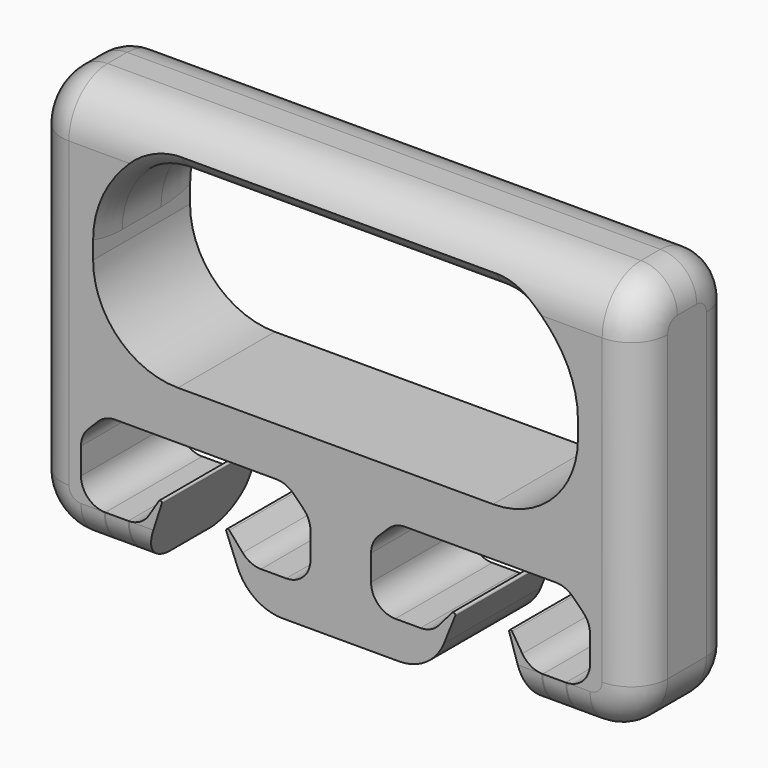
from build123d import *

# Parameters (mm, degrees)
F0_W        = 101.6
F0_H        = 38.1
F0_W_2      = 12.7
F0_H_2      = 7.6156796026
F1_DEPTH    = 25.4
F2_F1_R     = 0.3302
F2_F2_R     = 0.3302
F3_R        = 5.08
F5_R        = 10.15999
F6_T1_DEPTH = 101.6
F8_R        = 7.62
F9_W        = 12.7
F9_H        = 7.62
F10_DEPTH   = 25.4
F11_F1_R    = 0.381
F11_F2_R    = 0.381
F12_R       = 5.08
F13_SIZE    = 5.08
F14_R       = 5.08
F15_R       = 17.78
F16_R       = 10.16


# Not quite as in the source:
# - a fillet or chamfer that OpenCascade refuses, or shapes differently, is made with other operations: its cross-section is extruded or revolved along the edge and cut away or added
# - two fillets or chamfers of one size are made in one step
# - a fillet or chamfer is up to 0.001 mm smaller than in the source, because OpenCascade refuses the exact size


with BuildPart() as f1:
    # F0 (on Front) → F1 (new body)
    with BuildSketch(Plane.XZ):
        Polygon((63.5, 29.21), (-63.5, 29.21), (-63.5, -29.21), (-53.34, -29.21), (-5.08, -29.21), (-5.08, -29.2056796026), (5.08, -29.2056796026), (5.08, -29.21), (53.34, -29.21), (63.5, -29.21), align=None)
        Rectangle(F0_W, F0_H, mode=Mode.SUBTRACT)
        Polygon((63.5, -54.61), (63.5, -29.21), (53.34, -29.21), (53.34, -46.9943203974), (53.34, -54.61), align=None)
        with Locations((46.99, -50.8021601987)):
            Rectangle(F0_W_2, F0_H_2)
        Polygon((40.64, -54.61), (40.64, -46.9943203974), (35.5896614492, -38.9685556293), align=None)
        Polygon((-53.34, -29.21), (-63.5, -29.21), (-63.5, -54.61), (-53.34, -54.61), (-53.34, -46.9943203974), align=None)
        with Locations((-46.99, -50.8021601987)):
            Rectangle(F0_W_2, F0_H_2)
        Polygon((-35.5896614492, -38.9685556293), (-40.64, -46.9943203974), (-40.64, -54.61), align=None)
    extrude(amount=F1_DEPTH)

    # F2: fillet of radius 0.3302 on 2 edges, made by hand

    # F2_f1
    f2_f1_edges = [f1.edges().sort_by_distance(p)[0] for p in [
        (-35.5896614492, -12.7, -38.9685556293),
    ]]
    fillet(f2_f1_edges, radius=F2_F1_R)

    # F2_f2
    f2_f2_edges = [f1.edges().sort_by_distance(p)[0] for p in [
        (35.5896614492, -12.7, -38.9685556293),
    ]]
    fillet(f2_f2_edges, radius=F2_F2_R)

    # F3
    f3_edges = [f1.edges().sort_by_distance(p)[0] for p in [
        (53.34, -12.7, -46.99432),
        (-53.34, -12.7, -46.99432),
        (40.64, -12.7, -46.99432),
        (-40.64, -12.7, -46.99432),
    ]]
    fillet(f3_edges, radius=F3_R)

    # F5 (radius 10.16 in the source; OpenCascade refuses exactly that, so slightly less here)
    f5_edges = [f1.edges().sort_by_distance(p)[0] for p in [
        (-63.5, -12.7, -54.61),
        (63.5, -12.7, -54.61),
        (0, 0, 29.21),
        (0, -25.4, 29.21),
    ]]
    fillet(f5_edges, radius=F5_R)

    # F6: fillet of radius 7.62 on 2 edges, made by hand

    # F6_s2 → F6_t1 (cut)
    with BuildSketch(Plane.YZ.offset(-50.8)):
        with BuildLine():
            ThreePointArc((0, 26.67), (-2.2318463274, 21.2818463274), (-7.62, 19.05))
            Line((-7.62, 19.05), (0, 19.05))
            Line((0, 19.05), (0, 26.67))
        make_face()
        with BuildLine():
            ThreePointArc((-17.78, 19.05), (-23.1681536726, 21.2818463274), (-25.4, 26.67))
            Line((-25.4, 26.67), (-25.4, 19.05))
            Line((-25.4, 19.05), (-17.78, 19.05))
        make_face()
    extrude(amount=F6_T1_DEPTH, mode=Mode.SUBTRACT)

    # F8
    f8_edges = [f1.edges().sort_by_distance(p)[0] for p in [
        (-63.5, -25.4, -12.7),
        (-63.5, 0, -12.7),
        (63.5, 0, -12.7),
        (63.5, -25.4, -12.7),
        (46.990005, 0, -54.61),
        (60.524208, 0, -51.634208),
        (-60.524208, 0, -51.634208),
        (-46.990005, 0, -54.61),
        (46.990005, -25.4, -54.61),
        (60.524208, -25.4, -51.634208),
        (-60.524208, -25.4, -51.634208),
        (-46.990005, -25.4, -54.61),
        (-63.5, -22.424208, 26.234208),
        (63.5, -22.424208, 26.234208),
        (63.5, -12.7, 29.21),
        (-63.5, -12.7, 29.21),
        (-63.5, -2.975792, 26.234208),
        (63.5, -2.975792, 26.234208),
    ]]
    fillet(f8_edges, radius=F8_R)

    # F9 (on Front) → F10 (join)
    with BuildSketch(Plane.XZ):
        Polygon((7.4514560401, -29.0606748313), (-5.2485439599, -29.0606748313), (-5.2485439599, -46.8406748313), (-5.2485439599, -54.4606748313), (7.4514560401, -54.4606748313), (7.4514560401, -46.8406748313), (7.4514560401, -29.21), align=None)
        with Locations((-11.5985439599, -50.6506748313)):
            Rectangle(F9_W, F9_H)
        Polygon((-17.9485439599, -54.4606748313), (-17.9485439599, -46.8406748313), (-23.7521106244, -40.0734352433), align=None)
        with Locations((13.8014560401, -50.6506748313)):
            Rectangle(F9_W, F9_H)
        Polygon((25.9550227047, -40.0734352433), (20.1514560401, -46.8406748313), (20.1514560401, -54.4606748313), align=None)
    extrude(amount=F10_DEPTH)

    # F11: fillet of radius 0.381 on 2 edges, made by hand

    # F11_f1
    f11_f1_edges = [f1.edges().sort_by_distance(p)[0] for p in [
        (25.9550227047, -12.7, -40.0734352433),
    ]]
    fillet(f11_f1_edges, radius=F11_F1_R)

    # F11_f2
    f11_f2_edges = [f1.edges().sort_by_distance(p)[0] for p in [
        (-23.7521106244, -12.7, -40.0734352433),
    ]]
    fillet(f11_f2_edges, radius=F11_F2_R)

    # F12
    f12_edges = [f1.edges().sort_by_distance(p)[0] for p in [
        (-5.248544, -12.7, -46.840675),
        (7.451456, -12.7, -46.840675),
        (20.151456, -12.7, -46.840675),
        (-17.948544, -12.7, -46.840675),
    ]]
    fillet(f12_edges, radius=F12_R)

    # F13
    f13_edges = [f1.edges().sort_by_distance(p)[0] for p in [
        (7.451456, -12.7, -29.21),
        (-5.248544, -12.7, -29.21),
        (53.34, -12.7, -29.21),
        (-53.34, -12.7, -29.21),
    ]]
    chamfer(f13_edges, length=F13_SIZE)

    # F14
    f14_edges = [f1.edges().sort_by_distance(p)[0] for p in [
        (-53.34, -12.7, -34.29),
        (-48.26, -12.7, -29.21),
        (-10.328544, -12.7, -29.21),
        (-5.248544, -12.7, -34.29),
        (7.451456, -12.7, -34.29),
        (12.531456, -12.7, -29.21),
        (48.26, -12.7, -29.21),
        (53.34, -12.7, -34.29),
    ]]
    fillet(f14_edges, radius=F14_R)

    # F15 (call 1 of 4: OpenCascade refuses the feature's edges together)
    f15_edges = [f1.edges().sort_by_distance(p)[0] for p in [
        (-50.8, -12.7, 19.05),
    ]]
    fillet(f15_edges, radius=F15_R)

    # F15#3 (call 2 of 4)
    f15_3_edges = [f1.edges().sort_by_distance(p)[0] for p in [
        (-50.8, -12.7, -19.05),
    ]]
    fillet(f15_3_edges, radius=F15_R)

    # F15#4 (call 3 of 4)
    f15_4_edges = [f1.edges().sort_by_distance(p)[0] for p in [
        (50.8, -12.7, -19.05),
    ]]
    fillet(f15_4_edges, radius=F15_R)

    # F15#2 (call 4 of 4)
    f15_2_edges = [f1.edges().sort_by_distance(p)[0] for p in [
        (50.8, -12.7, 19.05),
    ]]
    fillet(f15_2_edges, radius=F15_R)

    # F16
    f16_edges = [f1.edges().sort_by_distance(p)[0] for p in [
        (-17.948544, -12.7, -54.460675),
        (20.151456, -12.7, -54.460675),
    ]]
    fillet(f16_edges, radius=F16_R)


solid = f1.part
